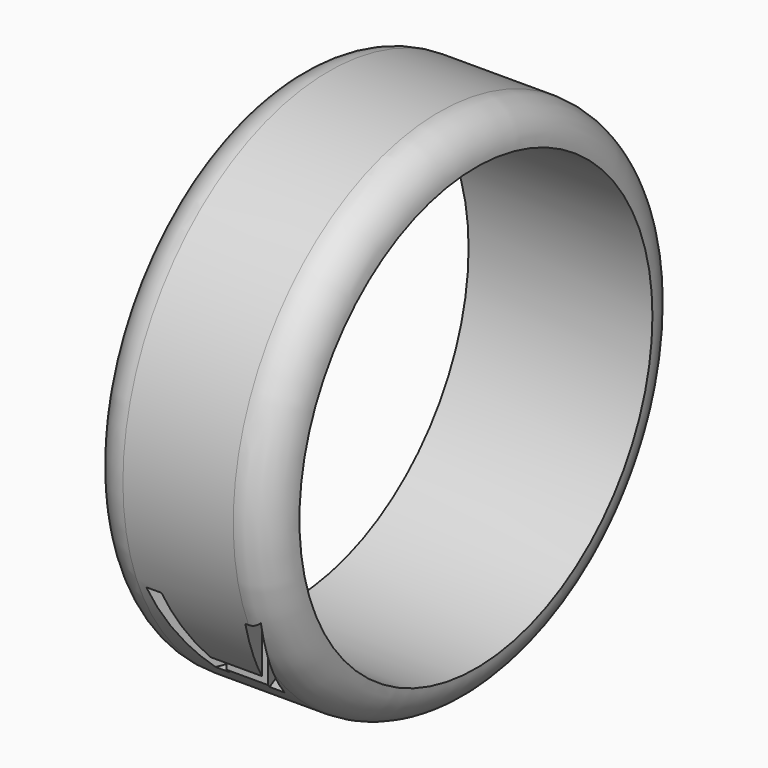
from build123d import *

# Parameters (mm, degrees)
F0_R         = 35
F0_R_2       = 30
F1_DEPTH     = 25
F2_R         = 4.99999
F3_TEXT_SIZE = 24.6050793471
F4_DEPTH     = 25


# Not quite as in the source:
# - a fillet or chamfer is up to 0.001 mm smaller than in the source, because OpenCascade refuses the exact size
# - Text() gives the source's letters only with a copy of the font that has no kerning and outlines rounded to 1/6400 em; it was checked with that copy


with BuildPart() as f1:
    # F0 (on Right) → F1 (new body)
    with BuildSketch(Plane.YZ):
        Circle(F0_R)
        Circle(F0_R_2, mode=Mode.SUBTRACT)
    extrude(amount=F1_DEPTH)

    # F2 (radius 5 in the source; OpenCascade refuses exactly that, so slightly less here)
    f2_edges = [f1.edges().sort_by_distance(p)[0] for p in [
        (12.5, 35, 0),
        (0, -35, 0),
        (25, -35, 0),
    ]]
    fillet(f2_edges, radius=F2_R)

    # F3 (on Top) → F4 (cut)
    with BuildSketch(Plane.XY):
        with Locations((6.0943309218, -32.3943458498)):
            Text('A', F3_TEXT_SIZE, font='Open Sans', text_align=(TextAlign.LEFT, TextAlign.BOTTOM))
    extrude(amount=-F4_DEPTH, mode=Mode.SUBTRACT)


solid = f1.part
